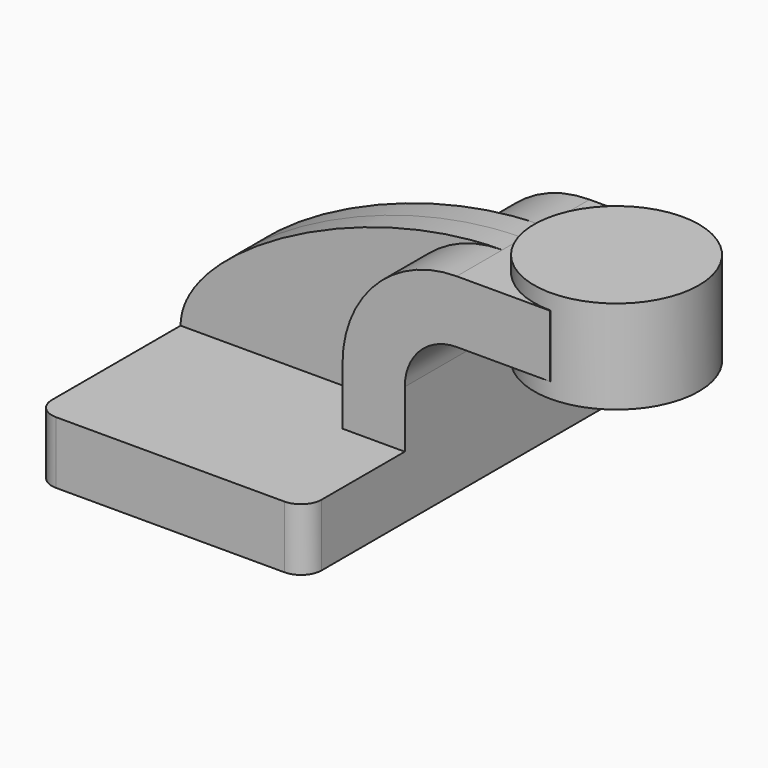
from build123d import *

# Parameters (mm, degrees)
F1_DEPTH = 63.5
F0_W     = 25.5854227781
F0_H     = 19.05
F2_DEPTH = 25.4
F3_DEPTH = 7.9375
F5_R     = 6.35


# Not quite as in the source:
# - a feature names something its author has since deleted; it is built from what else it names


with BuildPart() as f1:
    # F0 (on Front) → F1 (new body, symmetric)
    with BuildSketch(Plane.XZ):
        Polygon((22.225, 4.044502968), (-41.275, 4.044502968), (-41.275, -15.005497032), (41.275, -15.005497032), (41.275, 4.044502968), align=None)
    extrude(amount=F1_DEPTH, both=True)

    # F0 (on Front) → F2 (join, symmetric)
    with BuildSketch(Plane.XZ):
        with BuildLine():
            Line((22.225, 21.519702968), (22.225, 4.044502968))
            Line((22.225, 4.044502968), (41.275, 4.044502968))
            Line((41.275, 4.044502968), (41.275, 21.519702968))
            ThreePointArc((41.275, 21.519702968), (45.9246798487, 32.7450231193), (57.15, 37.394702968))
            Line((57.15, 37.394702968), (60.1395772219, 37.394702968))
            Line((60.1395772219, 37.394702968), (60.1395772219, 56.444702968))
            Line((60.1395772219, 56.444702968), (57.15, 56.444702968))
            ThreePointArc((57.15, 56.444702968), (32.4542956671, 46.2154073009), (22.225, 21.519702968))
        make_face()
        with Locations((72.9322886109, 46.919702968)):
            Rectangle(F0_W, F0_H)
    extrude(amount=F2_DEPTH, both=True)

    # F0 (on Front) → F3 (join, symmetric)
    with BuildSketch(Plane.XZ):
        with BuildLine():
            add(Edge.make_bspline(
                [(-41.275, 4.044502968), (-41.275, 26.4462009072), (13.2231097668, 56.444702968), (57.15, 56.444702968)],
                knots=[0, 0, 0, 0, 111.5045361635, 111.5045361635, 111.5045361635, 111.5045361635], degree=3))
            Line((-41.275, 4.044502968), (22.225, 4.044502968))
            Line((22.225, 4.044502968), (22.225, 21.519702968))
            ThreePointArc((22.225, 21.519702968), (32.4542956671, 46.2154073009), (57.15, 56.444702968))
        make_face()
    extrude(amount=F3_DEPTH, both=True)

    # F0 (on Front) → F4 (revolve)
    with BuildSketch(Plane.XZ):
        Polygon((85.725, 61.194502968), (85.725, 56.444702968), (85.725, 37.394702968), (85.725, 32.619502968), (110.9395772219, 32.619502968), (110.9395772219, 61.194502968), align=None)
    revolve(axis=Axis((85.725, 0, 46.907002968), (0, 0, -1)))

    # F5
    f5_edges = [f1.edges().sort_by_distance(p)[0] for p in [
        (-41.275, -63.5, -5.480497),
        (41.275, -63.5, -5.480497),
        (41.275, 63.5, -5.480497),
        (-41.275, 63.5, -5.480497),
    ]]
    fillet(f5_edges, radius=F5_R)


solid = f1.part
